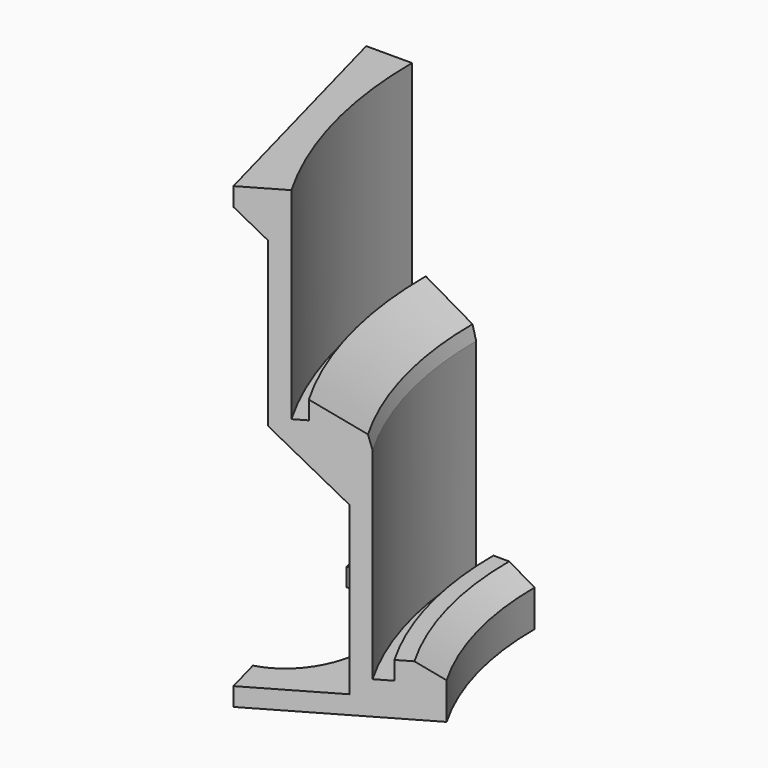
from build123d import *

# Parameters (mm, degrees)
F1_ANGLE = 30
F3_DEPTH = 25.4
F5_DEPTH = 25.4


with BuildPart() as f1:
    # F0 (on Front) → F1 (revolve)
    with BuildSketch(Plane.XZ):
        Polygon((-173.0375, 6.35), (-173.0375, 0), (-114.681, 0), (-114.681, 12.7), (-123.5075, 17.795982151), (-128.9685, 17.795982151), (-128.9685, 11.445982151), (-134.9375, 11.445982151), (-134.9375, 81.295982151), (-136.2075, 86.0356866766), (-152.4, 95.3844309105), (-152.4, 89.0344309105), (-157.1625, 89.0344309105), (-157.1625, 158.8844309105), (-173.0375, 158.8844309105), (-173.0375, 152.5344309105), (-163.5125, 143.0094309105), (-163.5125, 86.4041747894), (-141.2875, 64.1791747894), (-141.2875, 6.35), align=None)
    revolve(axis=Axis((0, 0, 96.6527089477), (0, 0, 1)), revolution_arc=F1_ANGLE)

    # F2 (on face) → F3 (cut)
    with BuildSketch(Plane(origin=(0, 0, 0), x_dir=(1, 0, 0), z_dir=(0, 0, -1))):
        with BuildLine():
            Line((-182.2236834316, 21.7005722844), (-168.6606251651, 72.3185948408))
            add(Edge.make_bspline(
                [(-168.6606251651, 72.3185948408), (-206.0052829566, 55.1989492048), (-182.2236834316, 21.7005722844)],
                knots=[0.5949234727, 0.5949234727, 0.5949234727, 2.5466691809, 2.5466691809, 2.5466691809], degree=2, weights=[1, 0.5604453769, 1]))
        make_face()
        with BuildLine():
            add(Edge.make_bspline(
                [(-143.5710023784, 68.2260600336), (-147.7895884166, 72.3535402758), (-153.2578255512, 73.81875)],
                knots=[5.8520567138, 5.8520567138, 5.8520567138, 6.2831853072, 6.2831853072, 6.2831853072], degree=2, weights=[1, 0.9768558474, 1]))
            Line((-153.2578255512, 73.81875), (-143.5710023784, 68.2260600336))
        make_face()
        with BuildLine():
            Line((-158.4491653232, 12.7), (-169.6345452561, 12.7))
            add(Edge.make_bspline(
                [(-169.6345452561, 12.7), (-164.1663081215, 11.2347902758), (-158.4491653232, 12.7)],
                knots=[3.1415926536, 3.1415926536, 3.1415926536, 3.572721247, 3.572721247, 3.572721247], degree=2, weights=[1, 0.9768558474, 1]))
        make_face()
        with BuildLine():
            Line((-143.5710023784, 68.2260600336), (-153.2578255512, 73.81875))
            Line((-153.2578255512, 73.81875), (-169.6345452561, 12.7))
            Line((-169.6345452561, 12.7), (-158.4491653232, 12.7))
            add(Edge.make_bspline(
                [(-158.4491653232, 12.7), (-141.7198075312, 16.987459415), (-136.4732452884, 36.5678954371)],
                knots=[3.572721247, 3.572721247, 3.572721247, 4.7123889674, 4.7123889674, 4.7123889674], degree=2, weights=[1, 0.8419906179, 1]))
            add(Edge.make_bspline(
                [(-136.4732452884, 36.5678954371), (-131.2266828952, 56.1483320204), (-143.5710023784, 68.2260600336)],
                knots=[4.7123889674, 4.7123889674, 4.7123889674, 5.8520567138, 5.8520567138, 5.8520567138], degree=2, weights=[1, 0.8419906109, 1]))
        make_face()
        with BuildLine():
            ThreePointArc((-173.0375, 0), (-172.9018353284, 6.8506748809), (-172.4950540409, 13.6906076446))
            add(Edge.make_bspline(
                [(-182.2236834316, 21.7005722844), (-178.3035736311, 16.1787689453), (-172.4950540409, 13.6906076446)],
                knots=[2.5466691809, 2.5466691809, 2.5466691809, 3.0245373947, 3.0245373947, 3.0245373947], degree=2, weights=[1, 0.9715907886, 1]))
            Line((-182.2236834316, 21.7005722844), (-188.0383342505, 0))
            Line((-188.0383342505, 0), (-173.0375, 0))
        make_face()
        with BuildLine():
            ThreePointArc((-156.2304026489, 74.391113007), (-153.1627191958, 80.5180591843), (-149.8548708073, 86.51875))
            Line((-149.8548708073, 86.51875), (-162.8085898503, 94.1586879635))
            Line((-162.8085898503, 94.1586879635), (-168.6606251651, 72.3185948408))
            add(Edge.make_bspline(
                [(-156.2304026489, 74.391113007), (-162.5048088227, 75.140561907), (-168.6606251651, 72.3185948408)],
                knots=[0.1170552589, 0.1170552589, 0.1170552589, 0.5949234727, 0.5949234727, 0.5949234727], degree=2, weights=[1, 0.9715907886, 1]))
        make_face()
        with BuildLine():
            Line((-153.2578255512, 73.81875), (-149.8548708073, 86.51875))
            ThreePointArc((-149.8548708073, 86.51875), (-153.1627191958, 80.5180591843), (-156.2304026489, 74.391113007))
            add(Edge.make_bspline(
                [(-153.2578255512, 73.81875), (-154.7211037363, 74.210834208), (-156.2304026489, 74.391113007)],
                knots=[0, 0, 0, 0.1170552589, 0.1170552589, 0.1170552589], degree=2, weights=[1, 0.9982877472, 1]))
        make_face()
        with BuildLine():
            Line((-173.0375, 0), (-169.6345452561, 12.7))
            add(Edge.make_bspline(
                [(-172.4950540409, 13.6906076446), (-171.0978234412, 13.092084208), (-169.6345452561, 12.7)],
                knots=[3.0245373947, 3.0245373947, 3.0245373947, 3.1415926536, 3.1415926536, 3.1415926536], degree=2, weights=[1, 0.9982877472, 1]))
            ThreePointArc((-172.4950540409, 13.6906076446), (-172.9018353284, 6.8506748809), (-173.0375, 0))
        make_face()
        with BuildLine():
            Line((-169.6345452561, 12.7), (-153.2578255512, 73.81875))
            add(Edge.make_bspline(
                [(-153.2578255512, 73.81875), (-154.7211037363, 74.210834208), (-156.2304026489, 74.391113007)],
                knots=[0, 0, 0, 0.1170552589, 0.1170552589, 0.1170552589], degree=2, weights=[1, 0.9982877472, 1]))
            ThreePointArc((-156.2304026489, 74.391113007), (-167.1413901665, 44.7854005169), (-172.4950540409, 13.6906076446))
            add(Edge.make_bspline(
                [(-172.4950540409, 13.6906076446), (-171.0978234412, 13.092084208), (-169.6345452561, 12.7)],
                knots=[3.0245373947, 3.0245373947, 3.0245373947, 3.1415926536, 3.1415926536, 3.1415926536], degree=2, weights=[1, 0.9982877472, 1]))
        make_face()
        with BuildLine():
            ThreePointArc((-172.4950540409, 13.6906076446), (-167.1413901665, 44.7854005169), (-156.2304026489, 74.391113007))
            add(Edge.make_bspline(
                [(-156.2304026489, 74.391113007), (-162.5048088227, 75.140561907), (-168.6606251651, 72.3185948408)],
                knots=[0.1170552589, 0.1170552589, 0.1170552589, 0.5949234727, 0.5949234727, 0.5949234727], degree=2, weights=[1, 0.9715907886, 1]))
            Line((-168.6606251651, 72.3185948408), (-182.2236834316, 21.7005722844))
            add(Edge.make_bspline(
                [(-182.2236834316, 21.7005722844), (-178.3035736311, 16.1787689453), (-172.4950540409, 13.6906076446)],
                knots=[2.5466691809, 2.5466691809, 2.5466691809, 3.0245373947, 3.0245373947, 3.0245373947], degree=2, weights=[1, 0.9715907886, 1]))
        make_face()
    extrude(amount=-F3_DEPTH, mode=Mode.SUBTRACT)

    # F4 (on face) → F5 (cut)
    with BuildSketch(Plane.XY.offset(158.8844309105)):
        Polygon((-149.8548708073, -86.51875), (-173.0375, 0), (-187.3384565115, -4.9058394507), (-165.3621643782, -86.51875), align=None)
    extrude(amount=-F5_DEPTH, mode=Mode.SUBTRACT)


solid = f1.part
